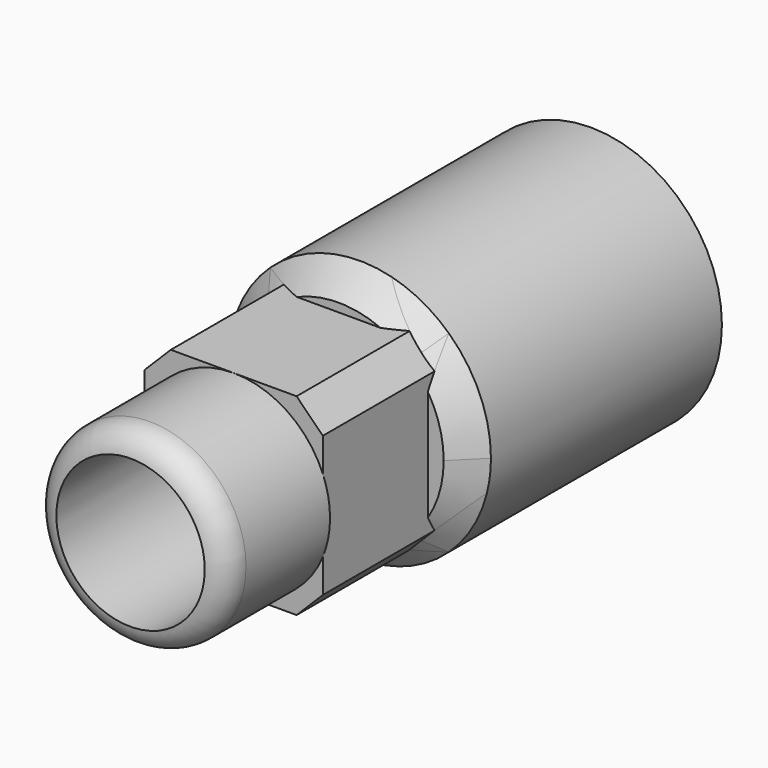
from build123d import *

# Parameters (mm, degrees)
F0_R         = 25
F1_DEPTH     = 60
F2_W         = 33.9622593881
F2_H         = 36.695571085
F3_DEPTH     = 25
F4_R         = 18.3477855425
F5_DEPTH     = 25.0000003725
F6_R         = 5
F8_T1_DEPTH  = 37.8584149398
F8_T6_ANGLE  = 94.4306250519
F8_T11_ANGLE = 94.4306250519
F8_T16_ANGLE = 94.4306250519
F8_T21_ANGLE = 47.2153125259
F8_T26_ANGLE = 47.2153125259
F8_T31_ANGLE = 47.2153125259
F8_T36_ANGLE = 47.2153125259
F8_T41_ANGLE = 85.5693749481
F8_T46_ANGLE = 85.5693749481
F8_T51_ANGLE = 85.5693749481
F8_T56_ANGLE = 85.5693749481
F8_T61_ANGLE = 85.5693749481
F8_T66_ANGLE = 85.5693749481
F9_R         = 14.0953649679
F10_DEPTH    = 200


# Not quite as in the source:
# - a fillet or chamfer that OpenCascade refuses, or shapes differently, is made with other operations: its cross-section is extruded or revolved along the edge and cut away or added
# - a feature of the source that left no trace in its solid (it failed there, or was rolled back) is left out


with BuildPart() as f1:
    # F0 (on Front) → F1 (new body)
    with BuildSketch(Plane.XZ):
        Circle(F0_R)
    extrude(amount=F1_DEPTH)

    # F2 (on face) → F3 (join)
    with BuildSketch(Plane.XZ.offset(60)):
        Rectangle(F2_W, F2_H)
    extrude(amount=F3_DEPTH)

    # F4 (on face) → F5 (join)
    with BuildSketch(Plane.XZ.offset(85)):
        Circle(F4_R)
    extrude(amount=F5_DEPTH)

    # F6
    f6_edges = [f1.edges().sort_by_distance(p)[0] for p in [
        (-18.347786, -110, 0),
    ]]
    fillet(f6_edges, radius=F6_R)

    # F8: chamfer of 5 on 9 edges, made by hand

    # F8_s2 → F8_t1 (cut)
    with BuildSketch(Plane.XZ.offset(60)):
        Polygon((16.9811296941, -13.3477855425), (11.9811296941, -18.3477855425), (16.9811296941, -18.3477855425), align=None)
        Polygon((16.9811296941, 13.3477855425), (11.9811296941, 18.3477855425), (16.9811296941, 18.3477855425), align=None)
        Polygon((-11.9811296941, -18.3477855425), (-16.9811296941, -13.3477855425), (-16.9811296941, -18.3477855425), align=None)
        Polygon((-16.9811296941, 13.3477855425), (-11.9811296941, 18.3477855425), (-16.9811296941, 18.3477855425), align=None)
    extrude(amount=F8_T1_DEPTH, mode=Mode.SUBTRACT)


with BuildPart() as f8_tool4:
    # F8_s5 → F8_t6 (revolve)
    with BuildSketch(Plane(origin=(0, 0, 0), x_dir=(0, 1, 0), z_dir=(0.7339114217, 0, 0.6792451878))):
        Polygon((-60, 20), (-55, 25), (-60, 25), align=None)
    revolve(axis=Axis((0, -60, 0), (0, -1, 0)), revolution_arc=F8_T6_ANGLE)

    split(bisect_by=Plane(origin=(-15.1644576183, 0, 15.1644576183), x_dir=(0, 1, 0), z_dir=(-0.7071067812, 0, 0.7071067812)), keep=Keep.TOP)


with BuildPart() as f1_1:
    add(f1.part)

    # F8_t3: cut F8_tool4
    add(f8_tool4.part, mode=Mode.SUBTRACT)


with BuildPart() as f8_tool9:
    # F8_s10 → F8_t11 (revolve)
    with BuildSketch(Plane(origin=(0, 0, 0), x_dir=(0, 1, 0), z_dir=(0.7339114217, 0, 0.6792451878))):
        Polygon((-60, 20), (-55, 25), (-60, 25), align=None)
    revolve(axis=Axis((0, -60, 0), (0, -1, 0)), revolution_arc=F8_T11_ANGLE)

    split(bisect_by=Plane.YZ.offset(-16.9811296941), keep=Keep.BOTTOM)


with BuildPart() as f1_2:
    add(f1_1.part)

    # F8_t8: cut F8_tool9
    add(f8_tool9.part, mode=Mode.SUBTRACT)


with BuildPart() as f8_tool14:
    # F8_s15 → F8_t16 (revolve)
    with BuildSketch(Plane(origin=(0, 0, 0), x_dir=(0, 1, 0), z_dir=(0.7339114217, 0, 0.6792451878))):
        Polygon((-60, 20), (-55, 25), (-60, 25), align=None)
    revolve(axis=Axis((0, -60, 0), (0, -1, 0)), revolution_arc=F8_T16_ANGLE)

    split(bisect_by=Plane(origin=(-15.1644576183, 0, -15.1644576183), x_dir=(0, 1, 0), z_dir=(-0.7071067812, 0, -0.7071067812)), keep=Keep.TOP)


with BuildPart() as f1_3:
    add(f1_2.part)

    # F8_t13: cut F8_tool14
    add(f8_tool14.part, mode=Mode.SUBTRACT)


with BuildPart() as f8_tool19:
    # F8_s20 → F8_t21 (revolve)
    with BuildSketch(Plane(origin=(0, 0, 0), x_dir=(0, 1, 0), z_dir=(-0.7339114217, 0, -0.6792451878))):
        Polygon((-60, 20), (-55, 25), (-60, 25), align=None)
    revolve(axis=Axis((0, -60, 0), (0, -1, 0)), revolution_arc=F8_T21_ANGLE)

    split(bisect_by=Plane(origin=(15.1644576183, 0, -15.1644576183), x_dir=(0, 1, 0), z_dir=(0.7071067812, 0, -0.7071067812)), keep=Keep.TOP)


with BuildPart() as f1_4:
    add(f1_3.part)

    # F8_t18: cut F8_tool19
    add(f8_tool19.part, mode=Mode.SUBTRACT)


with BuildPart() as f8_tool24:
    # F8_s25 → F8_t26 (revolve)
    with BuildSketch(Plane(origin=(0, 0, 0), x_dir=(0, 1, 0), z_dir=(-0.7339114217, 0, -0.6792451878))):
        Polygon((-60, 20), (-55, 25), (-60, 25), align=None)
    revolve(axis=Axis((0, -60, 0), (0, -1, 0)), revolution_arc=F8_T26_ANGLE)

    split(bisect_by=Plane.YZ.offset(16.9811296941), keep=Keep.TOP)


with BuildPart() as f1_5:
    add(f1_4.part)

    # F8_t23: cut F8_tool24
    add(f8_tool24.part, mode=Mode.SUBTRACT)


with BuildPart() as f8_tool29:
    # F8_s30 → F8_t31 (revolve)
    with BuildSketch(Plane.XY):
        Polygon((20, -60), (25, -55), (25, -60), align=None)
    revolve(axis=Axis((0, -60, 0), (0, -1, 0)), revolution_arc=F8_T31_ANGLE)

    split(bisect_by=Plane.YZ.offset(16.9811296941), keep=Keep.TOP)


with BuildPart() as f1_6:
    add(f1_5.part)

    # F8_t28: cut F8_tool29
    add(f8_tool29.part, mode=Mode.SUBTRACT)


with BuildPart() as f8_tool34:
    # F8_s35 → F8_t36 (revolve)
    with BuildSketch(Plane.XY):
        Polygon((20, -60), (25, -55), (25, -60), align=None)
    revolve(axis=Axis((0, -60, 0), (0, -1, 0)), revolution_arc=F8_T36_ANGLE)

    split(bisect_by=Plane(origin=(15.1644576183, 0, 15.1644576183), x_dir=(0, 1, 0), z_dir=(0.7071067812, 0, 0.7071067812)), keep=Keep.TOP)


with BuildPart() as f1_7:
    add(f1_6.part)

    # F8_t33: cut F8_tool34
    add(f8_tool34.part, mode=Mode.SUBTRACT)


with BuildPart() as f8_tool39:
    # F8_s40 → F8_t41 (revolve)
    with BuildSketch(Plane(origin=(0, 0, 0), x_dir=(0, 1, 0), z_dir=(-0.7339114217, 0, 0.6792451878))):
        Polygon((-60, 20), (-55, 25), (-60, 25), align=None)
    revolve(axis=Axis((0, -60, 0), (0, -1, 0)), revolution_arc=F8_T41_ANGLE)

    split(bisect_by=Plane(origin=(-15.1644576183, 0, -15.1644576183), x_dir=(0, 1, 0), z_dir=(-0.7071067812, 0, -0.7071067812)), keep=Keep.TOP)


with BuildPart() as f1_8:
    add(f1_7.part)

    # F8_t38: cut F8_tool39
    add(f8_tool39.part, mode=Mode.SUBTRACT)


with BuildPart() as f8_tool44:
    # F8_s45 → F8_t46 (revolve)
    with BuildSketch(Plane(origin=(0, 0, 0), x_dir=(0, 1, 0), z_dir=(-0.7339114217, 0, 0.6792451878))):
        Polygon((-60, 20), (-55, 25), (-60, 25), align=None)
    revolve(axis=Axis((0, -60, 0), (0, -1, 0)), revolution_arc=F8_T46_ANGLE)

    split(bisect_by=Plane.XY.offset(-18.3477855425), keep=Keep.BOTTOM)


with BuildPart() as f1_9:
    add(f1_8.part)

    # F8_t43: cut F8_tool44
    add(f8_tool44.part, mode=Mode.SUBTRACT)


with BuildPart() as f8_tool49:
    # F8_s50 → F8_t51 (revolve)
    with BuildSketch(Plane(origin=(0, 0, 0), x_dir=(0, 1, 0), z_dir=(-0.7339114217, 0, 0.6792451878))):
        Polygon((-60, 20), (-55, 25), (-60, 25), align=None)
    revolve(axis=Axis((0, -60, 0), (0, -1, 0)), revolution_arc=F8_T51_ANGLE)

    split(bisect_by=Plane(origin=(15.1644576183, 0, -15.1644576183), x_dir=(0, 1, 0), z_dir=(0.7071067812, 0, -0.7071067812)), keep=Keep.TOP)


with BuildPart() as f1_10:
    add(f1_9.part)

    # F8_t48: cut F8_tool49
    add(f8_tool49.part, mode=Mode.SUBTRACT)


with BuildPart() as f8_tool54:
    # F8_s55 → F8_t56 (revolve)
    with BuildSketch(Plane(origin=(0, 0, 0), x_dir=(0, 1, 0), z_dir=(0.7339114217, 0, -0.6792451878))):
        Polygon((-60, 20), (-55, 25), (-60, 25), align=None)
    revolve(axis=Axis((0, -60, 0), (0, -1, 0)), revolution_arc=F8_T56_ANGLE)

    split(bisect_by=Plane(origin=(15.1644576183, 0, 15.1644576183), x_dir=(0, 1, 0), z_dir=(0.7071067812, 0, 0.7071067812)), keep=Keep.TOP)


with BuildPart() as f1_11:
    add(f1_10.part)

    # F8_t53: cut F8_tool54
    add(f8_tool54.part, mode=Mode.SUBTRACT)


with BuildPart() as f8_tool59:
    # F8_s60 → F8_t61 (revolve)
    with BuildSketch(Plane(origin=(0, 0, 0), x_dir=(0, 1, 0), z_dir=(0.7339114217, 0, -0.6792451878))):
        Polygon((-60, 20), (-55, 25), (-60, 25), align=None)
    revolve(axis=Axis((0, -60, 0), (0, -1, 0)), revolution_arc=F8_T61_ANGLE)

    split(bisect_by=Plane.XY.offset(18.3477855425), keep=Keep.TOP)


with BuildPart() as f1_12:
    add(f1_11.part)

    # F8_t58: cut F8_tool59
    add(f8_tool59.part, mode=Mode.SUBTRACT)


with BuildPart() as f8_tool64:
    # F8_s65 → F8_t66 (revolve)
    with BuildSketch(Plane(origin=(0, 0, 0), x_dir=(0, 1, 0), z_dir=(0.7339114217, 0, -0.6792451878))):
        Polygon((-60, 20), (-55, 25), (-60, 25), align=None)
    revolve(axis=Axis((0, -60, 0), (0, -1, 0)), revolution_arc=F8_T66_ANGLE)

    split(bisect_by=Plane(origin=(-15.1644576183, 0, 15.1644576183), x_dir=(0, 1, 0), z_dir=(-0.7071067812, 0, 0.7071067812)), keep=Keep.TOP)


with BuildPart() as f1_13:
    add(f1_12.part)

    # F8_t63: cut F8_tool64
    add(f8_tool64.part, mode=Mode.SUBTRACT)

    # F9 (on face) → F10 (cut)
    with BuildSketch(Plane(origin=(0, 0, 0), x_dir=(-1, 0, 0), z_dir=(0, 1, 0))):
        with Locations((-0.2972558141, 0.1472756267)):
            Circle(F9_R)
    extrude(amount=-F10_DEPTH, mode=Mode.SUBTRACT)


solid = f1_13.part
